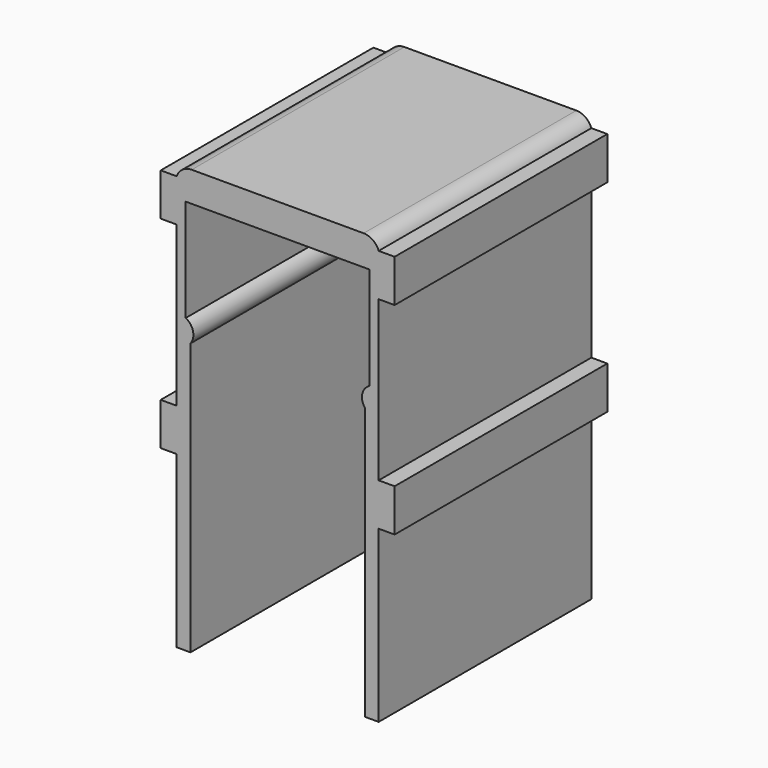
from build123d import *

# Parameters (mm, degrees)
F1_DEPTH    = 25
F2_T1_DEPTH = 32.0710678119


# Not quite as in the source:
# - a fillet or chamfer that OpenCascade refuses, or shapes differently, is made with other operations: its cross-section is extruded or revolved along the edge and cut away or added


with BuildPart() as f1:
    # F0 (on Front) → F1 (new body)
    with BuildSketch(Plane.XZ):
        with BuildLine():
            Line((9.5, 20), (0, 20))
            Line((0, 20), (0, 17.1773286244))
            Line((0, 17.1773286244), (8.65, 17.1773286244))
            Line((8.65, 17.1773286244), (8.65, 7.5421757065))
            ThreePointArc((8.65, 7.5421757065), (7.9600869661, 6.6679955593), (8.2, 5.5805156007))
            Line((8.2, 5.5805156007), (8.2, -20))
            Line((8.2, -20), (9.5, -20))
            Line((9.5, -20), (9.5, -4))
            Line((9.5, -4), (11, -4))
            Line((11, -4), (11, 0))
            Line((11, 0), (9.5, 0))
            Line((9.5, 0), (9.5, 15))
            Line((9.5, 15), (11, 15))
            Line((11, 15), (11, 19))
            Line((11, 19), (9.5, 19))
            Line((9.5, 19), (9.5, 20))
        make_face()
        with BuildLine():
            Line((0, 17.1773286244), (0, 20))
            Line((0, 20), (-9.5, 20))
            Line((-9.5, 20), (-9.5, 19))
            Line((-9.5, 19), (-11, 19))
            Line((-11, 19), (-11, 15))
            Line((-11, 15), (-9.5, 15))
            Line((-9.5, 15), (-9.5, 0))
            Line((-9.5, 0), (-11, 0))
            Line((-11, 0), (-11, -4))
            Line((-11, -4), (-9.5, -4))
            Line((-9.5, -4), (-9.5, -20))
            Line((-9.5, -20), (-8.2, -20))
            Line((-8.2, -20), (-8.2, 5.5805156007))
            ThreePointArc((-8.2, 5.5805156007), (-7.9600869661, 6.6679955593), (-8.65, 7.5421757065))
            Line((-8.65, 7.5421757065), (-8.65, 17.1773286244))
            Line((-8.65, 17.1773286244), (0, 17.1773286244))
        make_face()
    extrude(amount=F1_DEPTH)

    # F2: fillet of radius 1.5 on 2 edges, made by hand

    # F2_s2 → F2_t1 (cut)
    with BuildSketch(Plane.XZ.offset(-3.5355339059)):
        with BuildLine():
            ThreePointArc((-8.0857864376, 20), (-8.9518118414, 19.7247448714), (-9.5, 19))
            Line((-9.5, 19), (-9.5, 20))
            Line((-9.5, 20), (-8.0857864376, 20))
        make_face()
        with BuildLine():
            ThreePointArc((8.0857864376, 20), (8.9518118414, 19.7247448714), (9.5, 19))
            Line((9.5, 19), (9.5, 20))
            Line((9.5, 20), (8.0857864376, 20))
        make_face()
    extrude(amount=F2_T1_DEPTH, mode=Mode.SUBTRACT)


solid = f1.part
